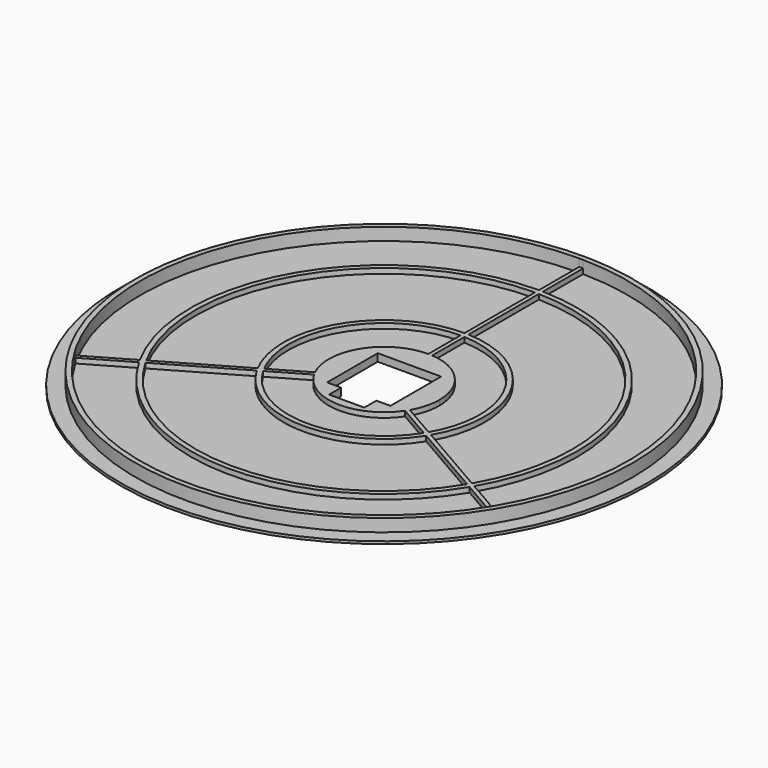
from build123d import *

# Parameters (mm, degrees)
F0_R     = 52.5
F0_R_2   = 49.5
F1_DEPTH = 0.5
F2_DEPTH = 3
F3_DEPTH = 1.5


# Not quite as in the source:
# - a feature names something its author has since deleted; it is built from what else it names


with BuildPart() as f1:
    # F0 (on Top) → F1 (new body)
    with BuildSketch(Plane.XY):
        Circle(F0_R)
        Circle(F0_R_2, mode=Mode.SUBTRACT)
        Circle(F0_R_2)
        with BuildLine():
            ThreePointArc((-42.3914543736, -23.5629920869), (-41.8034395488, 24.5911049344), (0, 48.5))
            Line((0, 48.5), (0.7895774504, 48.4935724344))
            ThreePointArc((0.7895774504, 48.4935724344), (42.1982413547, 23.9072881476), (42.0022320835, -24.25))
            Line((42.0022320835, -24.25), (41.6018769232, -24.9305803475))
            ThreePointArc((41.6018769232, -24.9305803475), (-0.3948018059, -48.498393082), (-42.0022320835, -24.25))
            Line((-42.0022320835, -24.25), (-42.3914543736, -23.5629920869))
        make_face(mode=Mode.SUBTRACT)
        with BuildLine():
            Line((0.7895774504, 48.4935724344), (0, 48.5))
            Line((0, 48.5), (0, 38.5))
            ThreePointArc((0, 38.5), (-33.1428201233, 19.5909028448), (-33.7297542357, -18.5621571806))
            Line((-33.7297542357, -18.5621571806), (-42.3914543736, -23.5629920869))
            Line((-42.3914543736, -23.5629920869), (-42.0022320835, -24.25))
            Line((-42.0022320835, -24.25), (-33.3419780457, -19.25))
            ThreePointArc((-33.3419780457, -19.25), (-0.394809485, -38.4979756022), (32.9401767853, -19.9297454412))
            Line((32.9401767853, -19.9297454412), (41.6018769232, -24.9305803475))
            Line((41.6018769232, -24.9305803475), (42.0022320835, -24.25))
            Line((42.0022320835, -24.25), (33.3419780457, -19.25))
            ThreePointArc((33.3419780457, -19.25), (33.5376296083, 18.9070727575), (0.7895774504, 38.4919026218))
            Line((0.7895774504, 38.4919026218), (0.7895774504, 48.4935724344))
        make_face()
        with BuildLine():
            ThreePointArc((32.0739643397, -19.4296374526), (-0.3948106071, -37.4979216035), (-32.4759526419, -18.75))
            Line((-32.4759526419, -18.75), (-17.3205080757, -10))
            ThreePointArc((-17.3205080757, -10), (-0.3948656915, -19.9961016472), (16.9122163764, -10.6759981846))
            Line((16.9122163764, -10.6759981846), (32.0739643397, -19.4296374526))
        make_face(mode=Mode.SUBTRACT)
        with BuildLine():
            Line((-17.7017938268, -9.308409924), (-32.8635417901, -18.0620491919))
            ThreePointArc((-32.8635417901, -18.0620491919), (-32.2767473942, 19.0908768172), (0, 37.5))
            Line((0, 37.5), (0, 20))
            ThreePointArc((0, 20), (-17.1196991574, 10.3400145435), (-17.7017938268, -9.308409924))
        make_face(mode=Mode.SUBTRACT)
        with BuildLine():
            ThreePointArc((0, 11), (0.3950435606, 10.9929041015), (0.7895774504, 10.971625561))
            Line((0.7895774504, 10.971625561), (0.7895774504, 18.983586791))
            ThreePointArc((0.7895774504, 18.983586791), (16.6483657305, 9.155977201), (16.4544826719, -9.5))
            Line((16.4544826719, -9.5), (9.5262794416, -5.5))
            ThreePointArc((9.5262794416, -5.5), (9.322612433, -5.8385698098), (9.1069177314, -6.1696069108))
            Line((9.1069177314, -6.1696069108), (16.0454796907, -10.1755875258))
            ThreePointArc((16.0454796907, -10.1755875258), (-0.3948740127, -18.9958962546), (-16.4544826719, -9.5))
            Line((-16.4544826719, -9.5), (-9.5262794416, -5.5))
            ThreePointArc((-9.5262794416, -5.5), (-9.7176559936, -5.1543342917), (-9.8964951818, -4.8020186502))
            Line((-9.8964951818, -4.8020186502), (-16.8350571411, -8.8079992652))
            ThreePointArc((-16.8350571411, -8.8079992652), (-16.2534917178, 9.8399190536), (0, 19))
            Line((0, 19), (0, 11))
        make_face(mode=Mode.SUBTRACT)
        with BuildLine():
            Line((32.4759526419, -18.75), (17.3205080757, -10))
            ThreePointArc((17.3205080757, -10), (17.5145648489, 9.6560871037), (0.7895774504, 19.9844081086))
            Line((0.7895774504, 19.9844081086), (0.7895774504, 37.4916866445))
            ThreePointArc((0.7895774504, 37.4916866445), (32.6715580013, 18.4070447863), (32.4759526419, -18.75))
        make_face(mode=Mode.SUBTRACT)
        with BuildLine():
            Line((-17.3205080757, -10), (-32.4759526419, -18.75))
            ThreePointArc((-32.4759526419, -18.75), (-0.3948106071, -37.4979216035), (32.0739643397, -19.4296374526))
            Line((32.0739643397, -19.4296374526), (16.9122163764, -10.6759981846))
            ThreePointArc((16.9122163764, -10.6759981846), (-0.3948656915, -19.9961016472), (-17.3205080757, -10))
        make_face()
        with BuildLine():
            ThreePointArc((0, 37.5), (-32.2767473942, 19.0908768172), (-32.8635417901, -18.0620491919))
            Line((-32.8635417901, -18.0620491919), (-17.7017938268, -9.308409924))
            ThreePointArc((-17.7017938268, -9.308409924), (-17.1196991574, 10.3400145435), (0, 20))
            Line((0, 20), (0, 37.5))
        make_face()
        with BuildLine():
            ThreePointArc((0.7895774504, 19.9844081086), (17.5145648489, 9.6560871037), (17.3205080757, -10))
            Line((17.3205080757, -10), (32.4759526419, -18.75))
            ThreePointArc((32.4759526419, -18.75), (32.6715580013, 18.4070447863), (0.7895774504, 37.4916866445))
            Line((0.7895774504, 37.4916866445), (0.7895774504, 19.9844081086))
        make_face()
        with BuildLine():
            Line((0, 38.5), (0, 48.5))
            ThreePointArc((0, 48.5), (-41.8034395488, 24.5911049344), (-42.3914543736, -23.5629920869))
            Line((-42.3914543736, -23.5629920869), (-33.7297542357, -18.5621571806))
            ThreePointArc((-33.7297542357, -18.5621571806), (-33.1428201233, 19.5909028448), (0, 38.5))
        make_face()
        with BuildLine():
            ThreePointArc((42.0022320835, -24.25), (42.1982413547, 23.9072881476), (0.7895774504, 48.4935724344))
            Line((0.7895774504, 48.4935724344), (0.7895774504, 38.4919026218))
            ThreePointArc((0.7895774504, 38.4919026218), (33.5376296083, 18.9070727575), (33.3419780457, -19.25))
            Line((33.3419780457, -19.25), (42.0022320835, -24.25))
        make_face()
        with BuildLine():
            Line((-33.3419780457, -19.25), (-42.0022320835, -24.25))
            ThreePointArc((-42.0022320835, -24.25), (-0.3948018059, -48.498393082), (41.6018769232, -24.9305803475))
            Line((41.6018769232, -24.9305803475), (32.9401767853, -19.9297454412))
            ThreePointArc((32.9401767853, -19.9297454412), (-0.394809485, -38.4979756022), (-33.3419780457, -19.25))
        make_face()
        with BuildLine():
            ThreePointArc((9.5262794416, -5.5), (10.6251840892, -2.8470094961), (11, 0))
            ThreePointArc((11, 0), (8.0524950157, 7.4938190546), (0.7895774504, 10.971625561))
            ThreePointArc((0.7895774504, 10.971625561), (0.3950435606, 10.9929041015), (0, 11))
            ThreePointArc((0, 11), (-9.322612433, 5.8385698098), (-9.8964951818, -4.8020186502))
            ThreePointArc((-9.8964951818, -4.8020186502), (-9.7176559936, -5.1543342917), (-9.5262794416, -5.5))
            ThreePointArc((-9.5262794416, -5.5), (-0.3950435606, -10.9929041015), (9.1069177314, -6.1696069108))
            ThreePointArc((9.1069177314, -6.1696069108), (9.322612433, -5.8385698098), (9.5262794416, -5.5))
        make_face()
        Polygon((6.3, 6.3), (6.3, -6.3), (3.5, -6.3), (3.5, -9.3), (-3.5, -9.3), (-3.5, -6.3), (-6.3, -6.3), (-6.3, 6.3), align=None, mode=Mode.SUBTRACT)
        with BuildLine():
            ThreePointArc((0.7895774504, 10.971625561), (8.0524950157, 7.4938190546), (11, 0))
            ThreePointArc((11, 0), (10.6251840892, -2.8470094961), (9.5262794416, -5.5))
            Line((9.5262794416, -5.5), (16.4544826719, -9.5))
            ThreePointArc((16.4544826719, -9.5), (16.6483657305, 9.155977201), (0.7895774504, 18.983586791))
            Line((0.7895774504, 18.983586791), (0.7895774504, 10.971625561))
        make_face()
        with BuildLine():
            ThreePointArc((-9.8964951818, -4.8020186502), (-9.322612433, 5.8385698098), (0, 11))
            Line((0, 11), (0, 19))
            ThreePointArc((0, 19), (-16.2534917178, 9.8399190536), (-16.8350571411, -8.8079992652))
            Line((-16.8350571411, -8.8079992652), (-9.8964951818, -4.8020186502))
        make_face()
        with BuildLine():
            Line((16.0454796907, -10.1755875258), (9.1069177314, -6.1696069108))
            ThreePointArc((9.1069177314, -6.1696069108), (-0.3950435606, -10.9929041015), (-9.5262794416, -5.5))
            Line((-9.5262794416, -5.5), (-16.4544826719, -9.5))
            ThreePointArc((-16.4544826719, -9.5), (-0.3948740127, -18.9958962546), (16.0454796907, -10.1755875258))
        make_face()
    extrude(amount=F1_DEPTH)

    # F0 (on Top) → F2 (join)
    with BuildSketch(Plane.XY):
        Circle(F0_R_2)
        with BuildLine():
            ThreePointArc((-42.3914543736, -23.5629920869), (-41.8034395488, 24.5911049344), (0, 48.5))
            Line((0, 48.5), (0.7895774504, 48.4935724344))
            ThreePointArc((0.7895774504, 48.4935724344), (42.1982413547, 23.9072881476), (42.0022320835, -24.25))
            Line((42.0022320835, -24.25), (41.6018769232, -24.9305803475))
            ThreePointArc((41.6018769232, -24.9305803475), (-0.3948018059, -48.498393082), (-42.0022320835, -24.25))
            Line((-42.0022320835, -24.25), (-42.3914543736, -23.5629920869))
        make_face(mode=Mode.SUBTRACT)
    extrude(amount=F2_DEPTH)

    # F0 (on Top) → F3 (join)
    with BuildSketch(Plane.XY):
        with BuildLine():
            Line((0.7895774504, 48.4935724344), (0, 48.5))
            Line((0, 48.5), (0, 38.5))
            ThreePointArc((0, 38.5), (-33.1428201233, 19.5909028448), (-33.7297542357, -18.5621571806))
            Line((-33.7297542357, -18.5621571806), (-42.3914543736, -23.5629920869))
            Line((-42.3914543736, -23.5629920869), (-42.0022320835, -24.25))
            Line((-42.0022320835, -24.25), (-33.3419780457, -19.25))
            ThreePointArc((-33.3419780457, -19.25), (-0.394809485, -38.4979756022), (32.9401767853, -19.9297454412))
            Line((32.9401767853, -19.9297454412), (41.6018769232, -24.9305803475))
            Line((41.6018769232, -24.9305803475), (42.0022320835, -24.25))
            Line((42.0022320835, -24.25), (33.3419780457, -19.25))
            ThreePointArc((33.3419780457, -19.25), (33.5376296083, 18.9070727575), (0.7895774504, 38.4919026218))
            Line((0.7895774504, 38.4919026218), (0.7895774504, 48.4935724344))
        make_face()
        with BuildLine():
            ThreePointArc((32.0739643397, -19.4296374526), (-0.3948106071, -37.4979216035), (-32.4759526419, -18.75))
            Line((-32.4759526419, -18.75), (-17.3205080757, -10))
            ThreePointArc((-17.3205080757, -10), (-0.3948656915, -19.9961016472), (16.9122163764, -10.6759981846))
            Line((16.9122163764, -10.6759981846), (32.0739643397, -19.4296374526))
        make_face(mode=Mode.SUBTRACT)
        with BuildLine():
            Line((-17.7017938268, -9.308409924), (-32.8635417901, -18.0620491919))
            ThreePointArc((-32.8635417901, -18.0620491919), (-32.2767473942, 19.0908768172), (0, 37.5))
            Line((0, 37.5), (0, 20))
            ThreePointArc((0, 20), (-17.1196991574, 10.3400145435), (-17.7017938268, -9.308409924))
        make_face(mode=Mode.SUBTRACT)
        with BuildLine():
            ThreePointArc((0, 11), (0.3950435606, 10.9929041015), (0.7895774504, 10.971625561))
            Line((0.7895774504, 10.971625561), (0.7895774504, 18.983586791))
            ThreePointArc((0.7895774504, 18.983586791), (16.6483657305, 9.155977201), (16.4544826719, -9.5))
            Line((16.4544826719, -9.5), (9.5262794416, -5.5))
            ThreePointArc((9.5262794416, -5.5), (9.322612433, -5.8385698098), (9.1069177314, -6.1696069108))
            Line((9.1069177314, -6.1696069108), (16.0454796907, -10.1755875258))
            ThreePointArc((16.0454796907, -10.1755875258), (-0.3948740127, -18.9958962546), (-16.4544826719, -9.5))
            Line((-16.4544826719, -9.5), (-9.5262794416, -5.5))
            ThreePointArc((-9.5262794416, -5.5), (-9.7176559936, -5.1543342917), (-9.8964951818, -4.8020186502))
            Line((-9.8964951818, -4.8020186502), (-16.8350571411, -8.8079992652))
            ThreePointArc((-16.8350571411, -8.8079992652), (-16.2534917178, 9.8399190536), (0, 19))
            Line((0, 19), (0, 11))
        make_face(mode=Mode.SUBTRACT)
        with BuildLine():
            Line((32.4759526419, -18.75), (17.3205080757, -10))
            ThreePointArc((17.3205080757, -10), (17.5145648489, 9.6560871037), (0.7895774504, 19.9844081086))
            Line((0.7895774504, 19.9844081086), (0.7895774504, 37.4916866445))
            ThreePointArc((0.7895774504, 37.4916866445), (32.6715580013, 18.4070447863), (32.4759526419, -18.75))
        make_face(mode=Mode.SUBTRACT)
        with BuildLine():
            ThreePointArc((9.5262794416, -5.5), (10.6251840892, -2.8470094961), (11, 0))
            ThreePointArc((11, 0), (8.0524950157, 7.4938190546), (0.7895774504, 10.971625561))
            ThreePointArc((0.7895774504, 10.971625561), (0.3950435606, 10.9929041015), (0, 11))
            ThreePointArc((0, 11), (-9.322612433, 5.8385698098), (-9.8964951818, -4.8020186502))
            ThreePointArc((-9.8964951818, -4.8020186502), (-9.7176559936, -5.1543342917), (-9.5262794416, -5.5))
            ThreePointArc((-9.5262794416, -5.5), (-0.3950435606, -10.9929041015), (9.1069177314, -6.1696069108))
            ThreePointArc((9.1069177314, -6.1696069108), (9.322612433, -5.8385698098), (9.5262794416, -5.5))
        make_face()
        Polygon((6.3, 6.3), (6.3, -6.3), (3.5, -6.3), (3.5, -9.3), (-3.5, -9.3), (-3.5, -6.3), (-6.3, -6.3), (-6.3, 6.3), align=None, mode=Mode.SUBTRACT)
    extrude(amount=F3_DEPTH)


solid = f1.part
